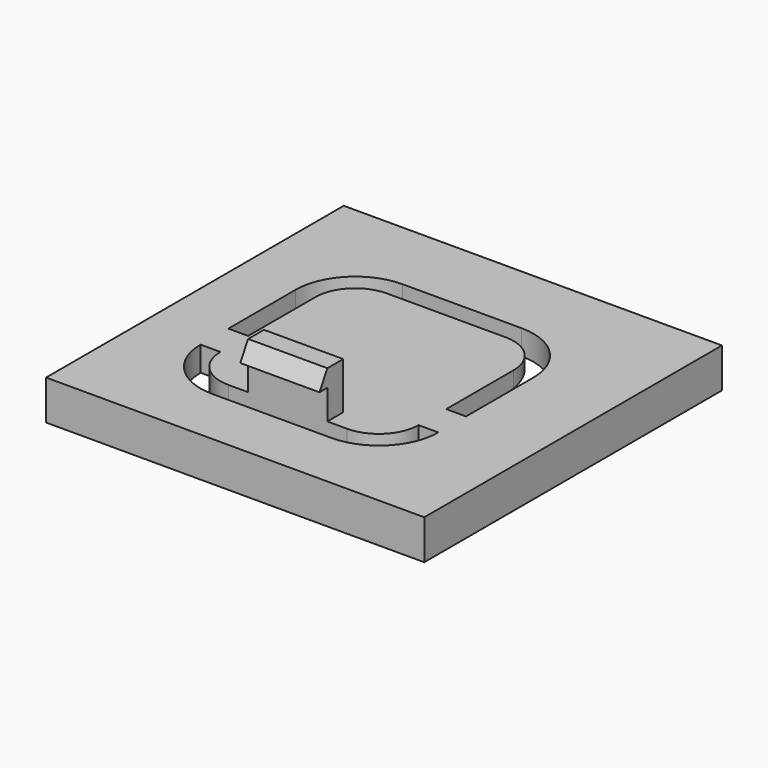
from build123d import *

# Parameters (mm, degrees)
F0_W        = 38.181103766
F0_H        = 37.5636257231
F1_DEPTH    = 2.5
F2_W        = 38.181103766
F2_H        = 37.5636257231
F2_W_2      = 32.181103766
F2_H_2      = 31.5636257231
F3_DEPTH    = 1.5
F5_DEPTH    = 22
F6_DEPTH    = 14
F7_T4_DEPTH = 63.9787194011


# Not quite as in the source:
# - a fillet or chamfer that OpenCascade refuses, or shapes differently, is made with other operations: its cross-section is extruded or revolved along the edge and cut away or added


with BuildPart() as f1:
    # F0 (on Top) → F1 (new body)
    with BuildSketch(Plane.XY):
        with Locations((19.090551883, 18.7818128616)):
            Rectangle(F0_W, F0_H)
        with BuildLine():
            ThreePointArc((8, 12), (9.1715728753, 9.1715728753), (12, 8))
            Line((12, 8), (24, 8))
            ThreePointArc((24, 8), (26.8284271247, 9.1715728753), (28, 12))
            Line((28, 12), (30, 12))
            ThreePointArc((30, 12), (28.2426406871, 7.7573593129), (24, 6))
            Line((24, 6), (12, 6))
            ThreePointArc((12, 6), (7.7573593129, 7.7573593129), (6, 12))
            Line((6, 12), (8, 12))
        make_face(mode=Mode.SUBTRACT)
        with BuildLine():
            Line((24, 28), (12, 28))
            ThreePointArc((12, 28), (9.1715728753, 26.8284271247), (8, 24))
            Line((8, 24), (8, 15.5))
            Line((8, 15.5), (6, 15.5))
            Line((6, 15.5), (6, 24))
            ThreePointArc((6, 24), (7.7573593129, 28.2426406871), (12, 30))
            Line((12, 30), (24, 30))
            ThreePointArc((24, 30), (28.2426406871, 28.2426406871), (30, 24))
            Line((30, 24), (30, 15.5))
            Line((30, 15.5), (28, 15.5))
            Line((28, 15.5), (28, 24))
            ThreePointArc((28, 24), (26.8284271247, 26.8284271247), (24, 28))
        make_face(mode=Mode.SUBTRACT)
    extrude(amount=F1_DEPTH)

    # F2 (on face) → F3 (join)
    with BuildSketch(Plane(origin=(0, 0, 0), x_dir=(1, 0, 0), z_dir=(0, 0, -1))):
        with Locations((19.090551883, -18.7818128616)):
            Rectangle(F2_W, F2_H)
        with Locations((19.090551883, -18.7818128616)):
            Rectangle(F2_W_2, F2_H_2, mode=Mode.SUBTRACT)
    extrude(amount=F3_DEPTH)

    # F4 (on Right) → F5 (join)
    with BuildSketch(Plane.YZ):
        Polygon((8, 5.5), (8, 2.5), (10, 2.5), (10, 7.2320508076), (8, 7.2320508076), (7, 5.5), align=None)
    extrude(amount=F5_DEPTH)

    # F4 (on Right) → F6 (cut)
    with BuildSketch(Plane.YZ):
        Polygon((8, 5.5), (8, 2.5), (10, 2.5), (10, 7.2320508076), (8, 7.2320508076), (7, 5.5), align=None)
    extrude(amount=F6_DEPTH, mode=Mode.SUBTRACT)

    # F7: chamfer of 10 x 1.5 on 1 edges, made by hand


with BuildPart() as f7_tool2:
    # F7_s3 → F7_t4 (new body)
    with BuildSketch(Plane.YZ.offset(49.9893597005)):
        Polygon((18, 0), (28, 1.5), (28, 0), align=None)
    extrude(amount=-F7_T4_DEPTH)

    split(bisect_by=Plane.YZ.offset(8), keep=Keep.TOP)

    split(bisect_by=Plane.YZ.offset(28), keep=Keep.BOTTOM)


with BuildPart() as f1_1:
    add(f1.part)

    # F7_t1: cut F7_tool2
    add(f7_tool2.part, mode=Mode.SUBTRACT)


solid = f1_1.part
